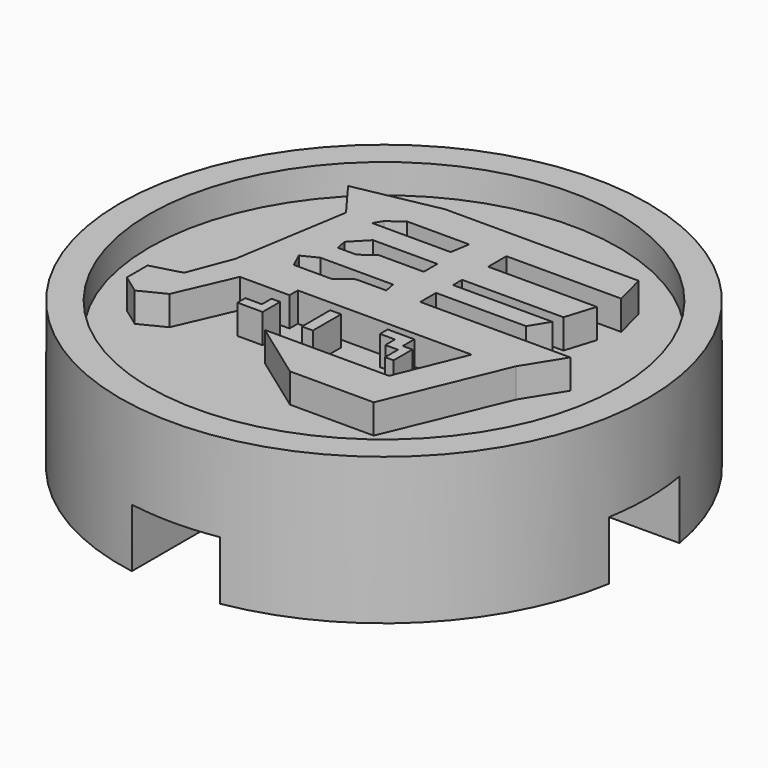
from build123d import *

# Parameters (mm, degrees)
F0_R     = 9
F1_DEPTH = 4
F2_W     = 3
F2_H     = 3
F3_DEPTH = 2
F5_R     = 9
F5_R_2   = 8
F5_W     = 0.3704614937
F5_H     = 1.2024026364
F4_DEPTH = 1


with BuildPart() as f1:
    # F0 (on Top) → F1 (new body)
    with BuildSketch(Plane.XY):
        with Locations((-31.3306450844, 19.7580661625)):
            Circle(F0_R)
    extrude(amount=F1_DEPTH)

    # F2 (on face) → F3 (cut)
    with BuildSketch(Plane(origin=(0, 0, 0), x_dir=(1, 0, 0), z_dir=(0, 0, -1))):
        with BuildLine():
            ThreePointArc((-32.8306450844, -28.6321858371), (-32.0832814269, -28.7265408676), (-31.3306450844, -28.7580661625))
            ThreePointArc((-31.3306450844, -28.7580661625), (-30.5780087419, -28.7265408676), (-29.8306450844, -28.6321858371))
            Line((-29.8306450844, -28.6321858371), (-29.8306450844, -21.2580661625))
            Line((-29.8306450844, -21.2580661625), (-32.8306450844, -21.2580661625))
            Line((-32.8306450844, -21.2580661625), (-32.8306450844, -28.6321858371))
        make_face()
        with BuildLine():
            ThreePointArc((-40.204764759, -18.2580661625), (-40.2991197895, -19.0054298199), (-40.3306450844, -19.7580661625))
            ThreePointArc((-40.3306450844, -19.7580661625), (-40.2991197895, -20.510702505), (-40.204764759, -21.2580661625))
            Line((-40.204764759, -21.2580661625), (-32.8306450844, -21.2580661625))
            Line((-32.8306450844, -21.2580661625), (-32.8306450844, -18.2580661625))
            Line((-32.8306450844, -18.2580661625), (-40.204764759, -18.2580661625))
        make_face()
        with Locations((-31.3306450844, -19.7580661625)):
            Rectangle(F2_W, F2_H)
        with BuildLine():
            Line((-29.8306450844, -18.2580661625), (-29.8306450844, -21.2580661625))
            Line((-29.8306450844, -21.2580661625), (-22.4565254097, -21.2580661625))
            ThreePointArc((-22.4565254097, -21.2580661625), (-22.3621703793, -20.510702505), (-22.3306450844, -19.7580661625))
            ThreePointArc((-22.3306450844, -19.7580661625), (-22.3621703793, -19.0054298199), (-22.4565254097, -18.2580661625))
            Line((-22.4565254097, -18.2580661625), (-29.8306450844, -18.2580661625))
        make_face()
        with BuildLine():
            Line((-32.8306450844, -10.8839464878), (-32.8306450844, -18.2580661625))
            Line((-32.8306450844, -18.2580661625), (-29.8306450844, -18.2580661625))
            Line((-29.8306450844, -18.2580661625), (-29.8306450844, -10.8839464878))
            ThreePointArc((-29.8306450844, -10.8839464878), (-30.5780087419, -10.7895914574), (-31.3306450844, -10.7580661625))
            ThreePointArc((-31.3306450844, -10.7580661625), (-32.0832814269, -10.7895914574), (-32.8306450844, -10.8839464878))
        make_face()
    extrude(amount=-F3_DEPTH, mode=Mode.SUBTRACT)

    # F5 (on face) → F4 (join)
    with BuildSketch(Plane.XY.offset(4)):
        with Locations((-31.3306450844, 19.7580661625)):
            Circle(F5_R)
        with Locations((-31.3306450844, 19.7580661625)):
            Circle(F5_R_2, mode=Mode.SUBTRACT)
        Polygon((-33.3540178835, 24.8932279646), (-36.2118817866, 24.328712374), (-35.2945402265, 23.0938345194), (-35.929620266, 19.1775020212), (-36.4941395819, 17.6956485957), (-37.51732409, 17.4133908004), (-37.51732409, 16.5313333273), (-36.8822440505, 16.0726644099), (-36.0354706645, 16.4960511029), (-35.1886935532, 18.4365753084), (-33.4951467812, 18.4365753084), (-33.4951467812, 18.7893975526), (-27.5677256286, 18.7893975526), (-28.5203475505, 16.4607688785), (-32.7542200685, 16.4607688785), (-30.7431295514, 15.0141958147), (-27.885267511, 15.0141958147), (-26.2270011008, 19.0010908991), (-25.4155080765, 20.3065350652), (-30.5314362049, 20.3065350652), (-30.5314362049, 20.9768973291), (-27.4618789554, 20.9768973291), (-27.0737744868, 21.6119792312), (-30.4608717561, 21.6119792312), (-30.4608717561, 22.0000836998), (-27.0032100379, 22.0000836998), (-26.6856700182, 23.0232700706), (-30.3903073072, 23.0232700706), (-30.3903073072, 23.7994790077), (-26.4739766717, 23.7994790077), (-26.756234467, 24.8932279646), align=None)
        Polygon((-34.499656409, 19.8707804084), (-34.7300246358, 20.377099514), (-34.2007912695, 20.6392026472), (-31.7267395564, 20.6392026472), (-31.6514596343, 20.258097545), (-32.6876805022, 20.258097545), (-33.209066838, 19.8707804084), align=None, mode=Mode.SUBTRACT)
        Polygon((-34.2753518545, 21.7523517899), (-33.7431058288, 22.3036166281), (-31.5476171672, 22.3036166281), (-31.5476171672, 21.7250771821), (-33.0903939903, 21.7250771821), (-33.5618001374, 21.3748883364), (-34.2007912695, 21.3748883364), align=None, mode=Mode.SUBTRACT)
        Polygon((-34.3772023916, 23.058552295), (-34.2007912695, 23.3408100903), (-33.7020926227, 23.7112734467), (-31.5899029374, 23.7112734467), (-31.6957496107, 23.058552295), align=None, mode=Mode.SUBTRACT)
        Polygon((-33.7434709072, 17.5698362291), (-34.3099012971, 17.5698362291), (-34.3099012971, 17.234172672), (-33.4497652948, 17.234172672), (-33.4497652948, 17.9789252579), (-33.7434709072, 17.9789252579), align=None)
        with Locations((-31.9214742631, 17.8353739902)):
            Rectangle(F5_W, F5_H)
        Polygon((-29.3105877936, 18.5256265104), (-30.2191060036, 18.5256265104), (-30.2191060036, 18.1992650032), (-29.707511887, 18.1992650032), (-29.707511887, 17.784697935), (-29.2753055692, 17.784697935), (-29.2753055692, 17.234172672), (-28.9842262864, 17.234172672), (-28.9842262864, 18.0316753685), (-29.3105877936, 18.0316753685), align=None)
    extrude(amount=F4_DEPTH)


solid = f1.part
